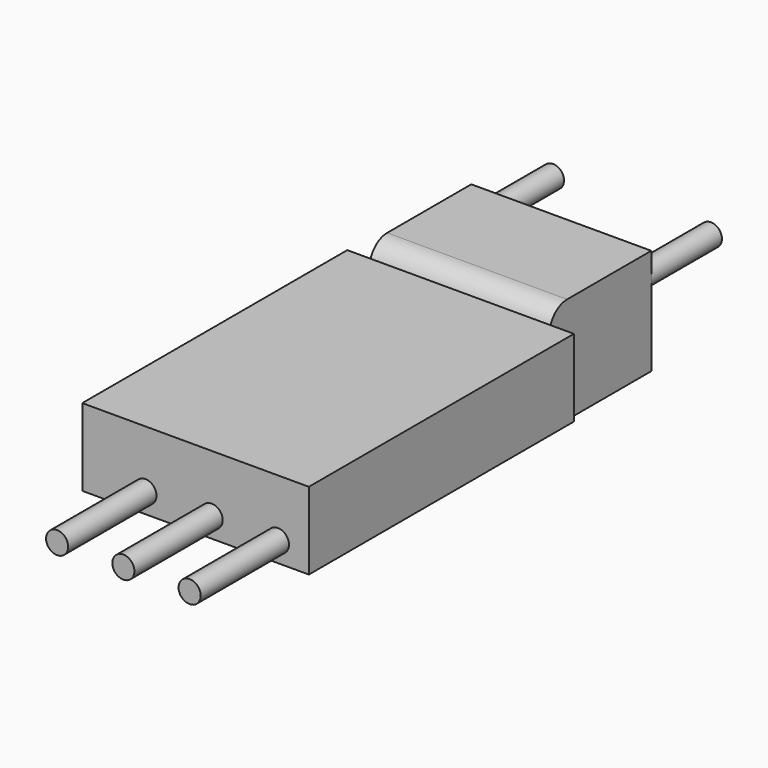
from build123d import *

# Parameters (mm, degrees)
F0_W        = 26.0604
F0_H        = 38.1
F1_DEPTH    = 4.445
F2_R        = 1.27
F3_DEPTH    = 12.7
F4_W        = 20.701
F4_H        = 12.192
F5_DEPTH    = 14.478
F6_R        = 1.27
F7_DEPTH    = 10.16
F6_R_2      = 0.635
F8_T1_DEPTH = 32.5977211869


# Not quite as in the source:
# - a fillet or chamfer that OpenCascade refuses, or shapes differently, is made with other operations: its cross-section is extruded or revolved along the edge and cut away or added


with BuildPart() as f1:
    # F0 (on Top) → F1 (new body, symmetric)
    with BuildSketch(Plane.XY):
        Rectangle(F0_W, F0_H)
    extrude(amount=F1_DEPTH, both=True)

    # F2 (on face) → F3 (join)
    with BuildSketch(Plane.XZ.offset(19.05)):
        with Locations((-5.7658, -2.159)):
            Circle(F2_R)
        with Locations((1.8542, -2.159)):
            Circle(F2_R)
        with Locations((9.4742, -2.159)):
            Circle(F2_R)
    extrude(amount=F3_DEPTH)

    # F4 (on face) → F5 (join)
    with BuildSketch(Plane(origin=(0, 19.05, 0), x_dir=(-1, 0, 0), z_dir=(0, 1, 0))):
        Rectangle(F4_W, F4_H)
    extrude(amount=F5_DEPTH)

    # F8: fillet of radius 2.54 on 2 edges, made by hand

    # F8_s2 → F8_t1 (cut)
    with BuildSketch(Plane.YZ.offset(-16.2988605935)):
        with BuildLine():
            ThreePointArc((19.05, 4.445), (19.9813214475, 5.6428229441), (21.4293442374, 6.096))
            Line((21.4293442374, 6.096), (19.05, 6.096))
            Line((19.05, 6.096), (19.05, 4.445))
        make_face()
        with BuildLine():
            ThreePointArc((19.05, -4.445), (19.9813214475, -5.6428229441), (21.4293442374, -6.096))
            Line((21.4293442374, -6.096), (19.05, -6.096))
            Line((19.05, -6.096), (19.05, -4.445))
        make_face()
    extrude(amount=F8_T1_DEPTH, mode=Mode.SUBTRACT)


with BuildPart() as f7:
    # F6 (on face) → F7 (new body)
    with BuildSketch(Plane(origin=(0, 33.528, 0), x_dir=(-1, 0, 0), z_dir=(0, 1, 0))):
        with Locations((-9.0805, 3.175)):
            Circle(F6_R)
    extrude(amount=F7_DEPTH)


with BuildPart() as f7b:
    # F6 (on face) → F7, piece 2 (new body)
    with BuildSketch(Plane(origin=(0, 33.528, 0), x_dir=(-1, 0, 0), z_dir=(0, 1, 0))):
        with Locations((9.0805, 3.175)):
            Circle(F6_R)
    extrude(amount=F7_DEPTH)


with BuildPart() as f7c:
    # F6 (on face) → F7, piece 3 (new body)
    with BuildSketch(Plane(origin=(0, 33.528, 0), x_dir=(-1, 0, 0), z_dir=(0, 1, 0))):
        with BuildLine():
            ThreePointArc((-0.635, -4.445), (0, -5.08), (0.635, -4.445))
            ThreePointArc((0.635, -4.445), (0, -3.81), (-0.635, -4.445))
        make_face()
    extrude(amount=F7_DEPTH)


with BuildPart() as f7d:
    # F6 (on face) → F7, piece 4 (new body)
    with BuildSketch(Plane(origin=(0, 33.528, 0), x_dir=(-1, 0, 0), z_dir=(0, 1, 0))):
        with Locations((-1.27, -4.445)):
            Circle(F6_R_2)
    extrude(amount=F7_DEPTH)


with BuildPart() as f7e:
    # F6 (on face) → F7, piece 5 (new body)
    with BuildSketch(Plane(origin=(0, 33.528, 0), x_dir=(-1, 0, 0), z_dir=(0, 1, 0))):
        with BuildLine():
            ThreePointArc((1.905, -4.445), (1.27, -3.81), (0.635, -4.445))
            ThreePointArc((0.635, -4.445), (1.27, -5.08), (1.905, -4.445))
        make_face()
    extrude(amount=F7_DEPTH)


solid = Compound([f1.part, f7.part, f7b.part, f7c.part, f7d.part, f7e.part])
